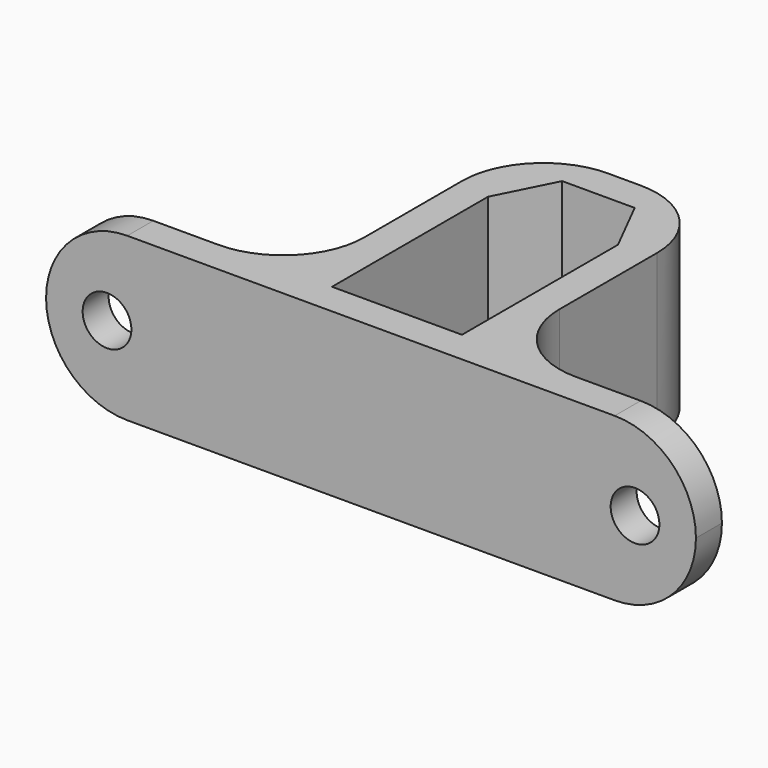
from build123d import *

# Parameters (mm, degrees)
F1_DEPTH = 10
F2_W     = 14
F2_H     = 2
F3_DEPTH = 10
F4_R     = 1.5
F5_DEPTH = 25
F6_R     = 4.99999


# Not quite as in the source:
# - a fillet or chamfer is up to 0.001 mm smaller than in the source, because OpenCascade refuses the exact size


with BuildPart() as f1:
    # F0 (on Top) → F1 (new body)
    with BuildSketch(Plane.XY):
        Polygon((4, 0), (0, 0), (-4, 0), (-6, 0), (-6, -2), (6, -2), (6, 0), align=None)
        Polygon((-6, 0), (-4, 0), (-4, 12), (-2.2325584196, 15.5), (2.2325584196, 15.5), (4, 12), (4, 0), (6, 0), (6, 17.5), (-6, 17.5), align=None)
    extrude(amount=F1_DEPTH)

    # F2 (on face) → F3 (join)
    with BuildSketch(Plane.XY.offset(10)):
        with Locations((-13, -1)):
            Rectangle(F2_W, F2_H)
        with Locations((13, -1)):
            Rectangle(F2_W, F2_H)
    extrude(amount=-F3_DEPTH)

    # F4 (on face) → F5 (cut)
    with BuildSketch(Plane(origin=(0, 0, 0), x_dir=(-1, 0, 0), z_dir=(0, 1, 0))):
        with Locations((16.25, 5)):
            Circle(F4_R)
        with Locations((-16.25, 5)):
            Circle(F4_R)
    extrude(amount=-F5_DEPTH, mode=Mode.SUBTRACT)

    # F6 (radius 5 in the source; OpenCascade refuses exactly that, so slightly less here)
    f6_edges = [f1.edges().sort_by_distance(p)[0] for p in [
        (-6, 17.5, 5),
        (6, 17.5, 5),
        (-6, 0, 5),
        (6, 0, 5),
        (-20, -1, 10),
        (-20, -1, 0),
        (20, -1, 10),
        (20, -1, 0),
    ]]
    fillet(f6_edges, radius=F6_R)


solid = f1.part
